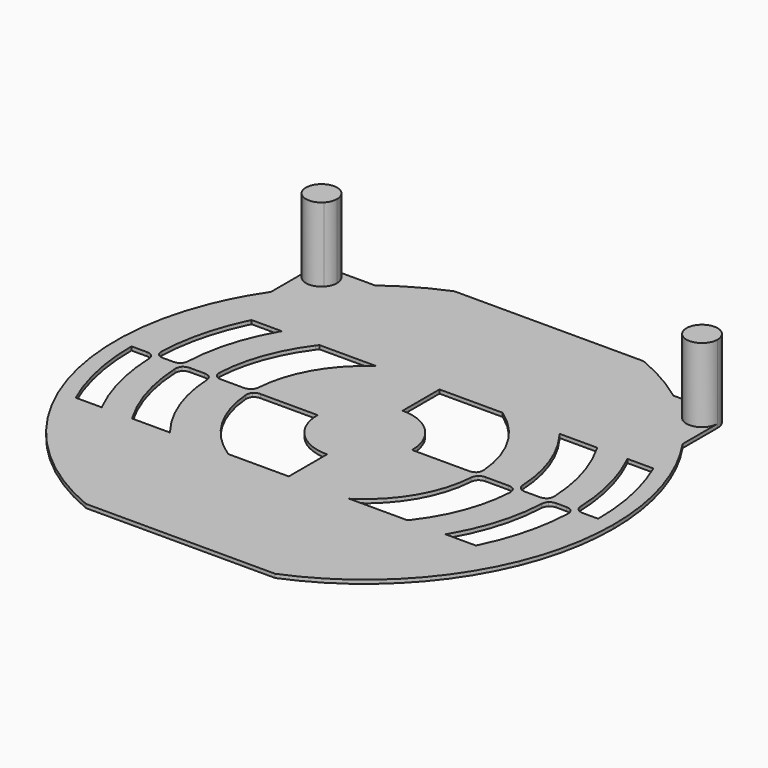
from build123d import *

# Parameters (mm, degrees)
F1_DEPTH    = 1.524
F2_T1_DEPTH = 1.524
F3_DEPTH    = 31.75
F5_DEPTH    = 12.7
F7_DEPTH    = 1.524


# Not quite as in the source:
# - a fillet or chamfer that OpenCascade refuses, or shapes differently, is made with other operations: its cross-section is extruded or revolved along the edge and cut away or added


with BuildPart() as f1:
    # F0 (on Top) → F1 (new body)
    with BuildSketch(Plane.XY):
        with BuildLine():
            ThreePointArc((-24.4320937034, 38.1), (-25.3223637573, 36.888098532), (-26.7450152278, 37.375283025))
            ThreePointArc((-26.7450152278, 37.375283025), (-40.5798224291, 21.5751160452), (-45.9412127468, 1.2698787713))
            ThreePointArc((-45.9412127468, 1.2698787713), (-45.0545517796, 0.8918001425), (-44.68876, 0))
            Line((-44.68876, 0), (-19.28622, 0))
            ThreePointArc((-19.28622, 0), (-13.6374169455, 13.6374169455), (0, 19.28622))
            Line((0, 19.28622), (0, 38.1))
            Line((0, 38.1), (-24.4320937034, 38.1))
        make_face()
        with BuildLine():
            ThreePointArc((25.7042798944, -38.0985251138), (40.2784862154, -22.1325816147), (45.9412127468, -1.2698787713))
            ThreePointArc((45.9412127468, -1.2698787713), (45.0545517796, -0.8918001425), (44.68876, 0))
            Line((44.68876, 0), (19.28622, 0))
            ThreePointArc((19.28622, 0), (13.6374169455, -13.6374169455), (0, -19.28622))
            Line((0, -19.28622), (0, -38.7942095688))
            Line((0, -38.7942095688), (23.3717719467, -38.7942095688))
            ThreePointArc((23.3717719467, -38.7942095688), (24.2787878517, -37.5771875695), (25.7042798944, -38.0985251138))
        make_face()
        with BuildLine():
            ThreePointArc((62.0544468751, 1.2699335332), (58.7091041954, 20.1397167987), (49.7668110589, 37.0895082899))
            ThreePointArc((49.7668110589, 37.0895082899), (48.4336499231, 36.9620417836), (47.7275214491, 38.1))
            Line((47.7275214491, 38.1), (26.9720937034, 38.1))
            ThreePointArc((26.9720937034, 38.1), (26.9139951713, 37.7202700539), (26.7450152278, 37.375283025))
            ThreePointArc((26.7450152278, 37.375283025), (40.5798224291, 21.5751160452), (45.9412127468, 1.2698787713))
            ThreePointArc((45.9412127468, 1.2698787713), (46.8505601425, 0.9042082204), (47.22876, 0))
            Line((47.22876, 0), (60.79744, 0))
            ThreePointArc((60.79744, 0), (61.1648323143, 0.8934200388), (62.0544468751, 1.2699335332))
        make_face()
        with BuildLine():
            ThreePointArc((64.5828161079, -37.7029056116), (72.0192608927, -20.1413824863), (74.7718960859, -1.2699542146))
            ThreePointArc((74.7718960859, -1.2699542146), (73.8808497579, -0.8942047945), (73.51268, 0))
            Line((73.51268, 0), (63.33744, 0))
            ThreePointArc((63.33744, 0), (62.9608600388, -0.9026076857), (62.0544468751, -1.2699335332))
            ThreePointArc((62.0544468751, -1.2699335332), (58.5641437485, -20.5574360064), (49.2333389626, -37.7947806284))
            ThreePointArc((49.2333389626, -37.7947806284), (49.5916770074, -38.238458905), (49.7197307741, -38.7942095688))
            Line((49.7197307741, -38.7942095688), (62.6632349558, -38.7942095688))
            ThreePointArc((62.6632349558, -38.7942095688), (63.3055678717, -37.6901561138), (64.5828161079, -37.7029056116))
        make_face()
        with BuildLine():
            ThreePointArc((85.6190619886, 1.2699650787), (83.3626938013, 19.5677762992), (77.2418743801, 36.9584825088))
            ThreePointArc((77.2418743801, 36.9584825088), (76.0121986911, 37.0230085698), (75.4152436073, 38.1))
            Line((75.4152436073, 38.1), (65.6193529725, 38.1))
            ThreePointArc((65.6193529725, 38.1), (65.4499936503, 37.4663675367), (64.9870851009, 37.0017296633))
            ThreePointArc((64.9870851009, 37.0017296633), (72.127201178, 19.7513563639), (74.7718960859, 1.2699542146))
            ThreePointArc((74.7718960859, 1.2699542146), (75.6768847945, 0.9018302421), (76.05268, 0))
            Line((76.05268, 0), (84.35848, 0))
            ThreePointArc((84.35848, 0), (84.7271307684, 0.8946896461), (85.6190619886, 1.2699650787))
        make_face()
        with BuildLine():
            ThreePointArc((93.901913207, -38.7942095688), (99.6568973575, -19.7753080655), (101.6, 0))
            Line((101.6, 0), (86.89848, 0))
            ThreePointArc((86.89848, 0), (86.5231696461, -0.9013492316), (85.6190619886, -1.2699650787))
            ThreePointArc((85.6190619886, -1.2699650787), (83.2730642114, -19.9457605507), (76.9033645528, -37.6577894674))
            ThreePointArc((76.9033645528, -37.6577894674), (77.4164332183, -38.1260574891), (77.6063995159, -38.7942095688))
            Line((77.6063995159, -38.7942095688), (93.901913207, -38.7942095688))
        make_face()
        with BuildLine():
            ThreePointArc((-60.79744, 0), (-61.1648323143, -0.8934200388), (-62.0544468751, -1.2699335332))
            ThreePointArc((-62.0544468751, -1.2699335332), (-58.5641437485, -20.5574360064), (-49.2333389626, -37.7947806284))
            ThreePointArc((-49.2333389626, -37.7947806284), (-47.8939801103, -37.6522633355), (-47.1797307741, -38.7942095688))
            Line((-47.1797307741, -38.7942095688), (-25.9117719467, -38.7942095688))
            ThreePointArc((-25.9117719467, -38.7942095688), (-25.858793946, -38.4312254739), (-25.7042798944, -38.0985251138))
            ThreePointArc((-25.7042798944, -38.0985251138), (-40.2784862154, -22.1325816147), (-45.9412127468, -1.2698787713))
            ThreePointArc((-45.9412127468, -1.2698787713), (-46.8505601425, -0.9042082204), (-47.22876, 0))
            Line((-47.22876, 0), (-60.79744, 0))
        make_face()
        with BuildLine():
            ThreePointArc((-62.6632349558, 38.1), (-63.4645367133, 36.9196517643), (-64.8572852825, 37.2287761518))
            ThreePointArc((-64.8572852825, 37.2287761518), (-72.0925536459, 19.8774479449), (-74.7718960859, 1.2699542146))
            ThreePointArc((-74.7718960859, 1.2699542146), (-73.8808497579, 0.8942047945), (-73.51268, 0))
            Line((-73.51268, 0), (-63.33744, 0))
            ThreePointArc((-63.33744, 0), (-62.9608600388, 0.9026076857), (-62.0544468751, 1.2699335332))
            ThreePointArc((-62.0544468751, 1.2699335332), (-58.7091041954, 20.1397167987), (-49.7668110589, 37.0895082899))
            ThreePointArc((-49.7668110589, 37.0895082899), (-50.1354796655, 37.536128474), (-50.2675214491, 38.1))
            Line((-50.2675214491, 38.1), (-62.6632349558, 38.1))
        make_face()
        with BuildLine():
            ThreePointArc((-84.35848, 0), (-84.7271307684, -0.8946896461), (-85.6190619886, -1.2699650787))
            ThreePointArc((-85.6190619886, -1.2699650787), (-83.2730642114, -19.9457605507), (-76.9033645528, -37.6577894674))
            ThreePointArc((-76.9033645528, -37.6577894674), (-75.6682474362, -37.7141758663), (-75.0663995159, -38.7942095688))
            Line((-75.0663995159, -38.7942095688), (-65.2032349558, -38.7942095688))
            ThreePointArc((-65.2032349558, -38.7942095688), (-65.0372884108, -38.1665424847), (-64.5828161079, -37.7029056116))
            ThreePointArc((-64.5828161079, -37.7029056116), (-72.0192608927, -20.1413824863), (-74.7718960859, -1.2699542146))
            ThreePointArc((-74.7718960859, -1.2699542146), (-75.6768847945, -0.9018302421), (-76.05268, 0))
            Line((-76.05268, 0), (-84.35848, 0))
        make_face()
        with BuildLine():
            Line((-77.9552436073, 38.1), (-94.1857207861, 38.1))
            ThreePointArc((-94.1857207861, 38.1), (-99.7292064339, 19.4073538656), (-101.6, 0))
            Line((-101.6, 0), (-86.89848, 0))
            ThreePointArc((-86.89848, 0), (-86.5231696461, 0.9013492316), (-85.6190619886, 1.2699650787))
            ThreePointArc((-85.6190619886, 1.2699650787), (-83.3626938013, 19.5677762992), (-77.2418743801, 36.9584825088))
            ThreePointArc((-77.2418743801, 36.9584825088), (-77.7622350375, 37.4269550838), (-77.9552436073, 38.1))
        make_face()
        with BuildLine():
            ThreePointArc((-85.6190619886, 1.2699650787), (-85.6261254648, 0.635), (-85.62848, 0))
            Line((-85.62848, 0), (-84.35848, 0))
            ThreePointArc((-84.35848, 0), (-84.7271307684, 0.8946896461), (-85.6190619886, 1.2699650787))
        make_face()
        with BuildLine():
            Line((-84.35848, 0), (-85.62848, 0))
            ThreePointArc((-85.62848, 0), (-85.6261254648, -0.635), (-85.6190619886, -1.2699650787))
            ThreePointArc((-85.6190619886, -1.2699650787), (-84.7271307684, -0.8946896461), (-84.35848, 0))
        make_face()
        with BuildLine():
            Line((-85.62848, 0), (-86.89848, 0))
            ThreePointArc((-86.89848, 0), (-86.5231696461, -0.9013492316), (-85.6190619886, -1.2699650787))
            ThreePointArc((-85.6190619886, -1.2699650787), (-85.6261254648, -0.635), (-85.62848, 0))
        make_face()
        with BuildLine():
            ThreePointArc((-85.6190619886, 1.2699650787), (-86.5231696461, 0.9013492316), (-86.89848, 0))
            Line((-86.89848, 0), (-85.62848, 0))
            ThreePointArc((-85.62848, 0), (-85.6261254648, 0.635), (-85.6190619886, 1.2699650787))
        make_face()
        with BuildLine():
            ThreePointArc((-74.7718960859, 1.2699542146), (-75.6768847945, 0.9018302421), (-76.05268, 0))
            Line((-76.05268, 0), (-74.78268, 0))
            ThreePointArc((-74.78268, 0), (-74.7799839729, 0.635), (-74.7718960859, 1.2699542146))
        make_face()
        with BuildLine():
            ThreePointArc((-74.7718960859, 1.2699542146), (-74.7799839729, 0.635), (-74.78268, 0))
            Line((-74.78268, 0), (-73.51268, 0))
            ThreePointArc((-73.51268, 0), (-73.8808497579, 0.8942047945), (-74.7718960859, 1.2699542146))
        make_face()
        with BuildLine():
            Line((-73.51268, 0), (-74.78268, 0))
            ThreePointArc((-74.78268, 0), (-74.7799839729, -0.635), (-74.7718960859, -1.2699542146))
            ThreePointArc((-74.7718960859, -1.2699542146), (-73.8808497579, -0.8942047945), (-73.51268, 0))
        make_face()
        with BuildLine():
            Line((-74.78268, 0), (-76.05268, 0))
            ThreePointArc((-76.05268, 0), (-75.6768847945, -0.9018302421), (-74.7718960859, -1.2699542146))
            ThreePointArc((-74.7718960859, -1.2699542146), (-74.7799839729, -0.635), (-74.78268, 0))
        make_face()
        with BuildLine():
            ThreePointArc((-62.0544468751, 1.2699335332), (-62.9608600388, 0.9026076857), (-63.33744, 0))
            Line((-63.33744, 0), (-62.06744, 0))
            ThreePointArc((-62.06744, 0), (-62.0641916338, 0.635), (-62.0544468751, 1.2699335332))
        make_face()
        with BuildLine():
            ThreePointArc((-62.0544468751, 1.2699335332), (-62.0641916338, 0.635), (-62.06744, 0))
            Line((-62.06744, 0), (-60.79744, 0))
            ThreePointArc((-60.79744, 0), (-61.1648323143, 0.8934200388), (-62.0544468751, 1.2699335332))
        make_face()
        with BuildLine():
            Line((-60.79744, 0), (-62.06744, 0))
            ThreePointArc((-62.06744, 0), (-62.0641916338, -0.635), (-62.0544468751, -1.2699335332))
            ThreePointArc((-62.0544468751, -1.2699335332), (-61.1648323143, -0.8934200388), (-60.79744, 0))
        make_face()
        with BuildLine():
            Line((-62.06744, 0), (-63.33744, 0))
            ThreePointArc((-63.33744, 0), (-62.9608600388, -0.9026076857), (-62.0544468751, -1.2699335332))
            ThreePointArc((-62.0544468751, -1.2699335332), (-62.0641916338, -0.635), (-62.06744, 0))
        make_face()
        with BuildLine():
            ThreePointArc((-45.9412127468, 1.2698787713), (-46.8505601425, 0.9042082204), (-47.22876, 0))
            Line((-47.22876, 0), (-45.95876, 0))
            ThreePointArc((-45.95876, 0), (-45.9543729773, 0.635), (-45.9412127468, 1.2698787713))
        make_face()
        with BuildLine():
            ThreePointArc((-45.9412127468, 1.2698787713), (-45.9543729773, 0.635), (-45.95876, 0))
            Line((-45.95876, 0), (-44.68876, 0))
            ThreePointArc((-44.68876, 0), (-45.0545517796, 0.8918001425), (-45.9412127468, 1.2698787713))
        make_face()
        with BuildLine():
            Line((-44.68876, 0), (-45.95876, 0))
            ThreePointArc((-45.95876, 0), (-45.9543729773, -0.635), (-45.9412127468, -1.2698787713))
            ThreePointArc((-45.9412127468, -1.2698787713), (-45.0545517796, -0.8918001425), (-44.68876, 0))
        make_face()
        with BuildLine():
            Line((-45.95876, 0), (-47.22876, 0))
            ThreePointArc((-47.22876, 0), (-46.8505601425, -0.9042082204), (-45.9412127468, -1.2698787713))
            ThreePointArc((-45.9412127468, -1.2698787713), (-45.9543729773, -0.635), (-45.95876, 0))
        make_face()
        with BuildLine():
            ThreePointArc((45.9412127468, -1.2698787713), (46.8505601425, -0.9042082204), (47.22876, 0))
            Line((47.22876, 0), (45.95876, 0))
            ThreePointArc((45.95876, 0), (45.9543729773, -0.635), (45.9412127468, -1.2698787713))
        make_face()
        with BuildLine():
            Line((45.95876, 0), (47.22876, 0))
            ThreePointArc((47.22876, 0), (46.8505601425, 0.9042082204), (45.9412127468, 1.2698787713))
            ThreePointArc((45.9412127468, 1.2698787713), (45.9543729773, 0.635), (45.95876, 0))
        make_face()
        with BuildLine():
            Line((44.68876, 0), (45.95876, 0))
            ThreePointArc((45.95876, 0), (45.9543729773, 0.635), (45.9412127468, 1.2698787713))
            ThreePointArc((45.9412127468, 1.2698787713), (45.0545517796, 0.8918001425), (44.68876, 0))
        make_face()
        with BuildLine():
            Line((60.79744, 0), (62.06744, 0))
            ThreePointArc((62.06744, 0), (62.0641916338, 0.635), (62.0544468751, 1.2699335332))
            ThreePointArc((62.0544468751, 1.2699335332), (61.1648323143, 0.8934200388), (60.79744, 0))
        make_face()
        with BuildLine():
            Line((62.06744, 0), (63.33744, 0))
            ThreePointArc((63.33744, 0), (62.9608600388, 0.9026076857), (62.0544468751, 1.2699335332))
            ThreePointArc((62.0544468751, 1.2699335332), (62.0641916338, 0.635), (62.06744, 0))
        make_face()
        with BuildLine():
            ThreePointArc((62.0544468751, -1.2699335332), (62.9608600388, -0.9026076857), (63.33744, 0))
            Line((63.33744, 0), (62.06744, 0))
            ThreePointArc((62.06744, 0), (62.0641916338, -0.635), (62.0544468751, -1.2699335332))
        make_face()
        with BuildLine():
            ThreePointArc((62.0544468751, -1.2699335332), (62.0641916338, -0.635), (62.06744, 0))
            Line((62.06744, 0), (60.79744, 0))
            ThreePointArc((60.79744, 0), (61.1648323143, -0.8934200388), (62.0544468751, -1.2699335332))
        make_face()
        with BuildLine():
            Line((73.51268, 0), (74.78268, 0))
            ThreePointArc((74.78268, 0), (74.7799839729, 0.635), (74.7718960859, 1.2699542146))
            ThreePointArc((74.7718960859, 1.2699542146), (73.8808497579, 0.8942047945), (73.51268, 0))
        make_face()
        with BuildLine():
            ThreePointArc((74.7718960859, -1.2699542146), (74.7799839729, -0.635), (74.78268, 0))
            Line((74.78268, 0), (73.51268, 0))
            ThreePointArc((73.51268, 0), (73.8808497579, -0.8942047945), (74.7718960859, -1.2699542146))
        make_face()
        with BuildLine():
            ThreePointArc((74.7718960859, -1.2699542146), (75.6768847945, -0.9018302421), (76.05268, 0))
            Line((76.05268, 0), (74.78268, 0))
            ThreePointArc((74.78268, 0), (74.7799839729, -0.635), (74.7718960859, -1.2699542146))
        make_face()
        with BuildLine():
            Line((74.78268, 0), (76.05268, 0))
            ThreePointArc((76.05268, 0), (75.6768847945, 0.9018302421), (74.7718960859, 1.2699542146))
            ThreePointArc((74.7718960859, 1.2699542146), (74.7799839729, 0.635), (74.78268, 0))
        make_face()
        with BuildLine():
            Line((84.35848, 0), (85.62848, 0))
            ThreePointArc((85.62848, 0), (85.6261254648, 0.635), (85.6190619886, 1.2699650787))
            ThreePointArc((85.6190619886, 1.2699650787), (84.7271307684, 0.8946896461), (84.35848, 0))
        make_face()
        with BuildLine():
            Line((85.62848, 0), (86.89848, 0))
            ThreePointArc((86.89848, 0), (86.5231696461, 0.9013492316), (85.6190619886, 1.2699650787))
            ThreePointArc((85.6190619886, 1.2699650787), (85.6261254648, 0.635), (85.62848, 0))
        make_face()
        with BuildLine():
            ThreePointArc((85.6190619886, -1.2699650787), (86.5231696461, -0.9013492316), (86.89848, 0))
            Line((86.89848, 0), (85.62848, 0))
            ThreePointArc((85.62848, 0), (85.6261254648, -0.635), (85.6190619886, -1.2699650787))
        make_face()
        with BuildLine():
            ThreePointArc((85.6190619886, -1.2699650787), (85.6261254648, -0.635), (85.62848, 0))
            Line((85.62848, 0), (84.35848, 0))
            ThreePointArc((84.35848, 0), (84.7271307684, -0.8946896461), (85.6190619886, -1.2699650787))
        make_face()
        with BuildLine():
            Line((0, 0), (0, 19.28622))
            ThreePointArc((0, 19.28622), (-13.6374169455, 13.6374169455), (-19.28622, 0))
            Line((-19.28622, 0), (0, 0))
        make_face()
        with BuildLine():
            Line((0, 0), (19.28622, 0))
            ThreePointArc((19.28622, 0), (13.6374169455, 13.6374169455), (0, 19.28622))
            Line((0, 19.28622), (0, 0))
        make_face()
        with BuildLine():
            ThreePointArc((0, -19.28622), (13.6374169455, -13.6374169455), (19.28622, 0))
            Line((19.28622, 0), (0, 0))
            Line((0, 0), (0, -19.28622))
        make_face()
        with BuildLine():
            Line((0, 0), (-19.28622, 0))
            ThreePointArc((-19.28622, 0), (-13.6374169455, -13.6374169455), (0, -19.28622))
            Line((0, -19.28622), (0, 0))
        make_face()
        with BuildLine():
            ThreePointArc((45.9412127468, -1.2698787713), (45.9543729773, -0.635), (45.95876, 0))
            Line((45.95876, 0), (44.68876, 0))
            ThreePointArc((44.68876, 0), (45.0545517796, -0.8918001425), (45.9412127468, -1.2698787713))
        make_face()
        with BuildLine():
            ThreePointArc((73.0914093882, 70.5705737092), (67.2072279768, 76.1954625137), (60.8916274027, 81.3312345428))
            ThreePointArc((60.8916274027, 81.3312345428), (0, 101.6), (-60.8916274027, 81.3312345428))
            ThreePointArc((-60.8916274027, 81.3312345428), (-67.2072281578, 76.195462354), (-73.0914097236, 70.5705733618))
            ThreePointArc((-73.0914097236, 70.5705733618), (-78.8370521258, 64.0880582646), (-84.0096224974, 57.1396826019))
            ThreePointArc((-84.0096224974, 57.1396826019), (-89.6048127635, 47.8908919276), (-94.1857207861, 38.1))
            Line((-94.1857207861, 38.1), (-77.9552436073, 38.1))
            ThreePointArc((-77.9552436073, 38.1), (-77.35028331, 39.1819529536), (-76.1117440894, 39.2331364891))
            ThreePointArc((-76.1117440894, 39.2331364891), (0, 85.62848), (76.1117440894, 39.2331364891))
            ThreePointArc((76.1117440894, 39.2331364891), (77.35028331, 39.1819529536), (77.9552436073, 38.1))
            Line((77.9552436073, 38.1), (94.1857207861, 38.1))
            ThreePointArc((94.1857207861, 38.1), (89.6048127635, 47.8908919276), (84.0096224974, 57.1396826019))
            ThreePointArc((84.0096224974, 57.1396826019), (78.8370519734, 64.0880584519), (73.0914093882, 70.5705737092))
        make_face()
        with BuildLine():
            ThreePointArc((75.4152436073, 38.1), (75.6032906537, 38.7650397027), (76.1117440894, 39.2331364891))
            ThreePointArc((76.1117440894, 39.2331364891), (0, 85.62848), (-76.1117440894, 39.2331364891))
            ThreePointArc((-76.1117440894, 39.2331364891), (-75.6032906537, 38.7650397027), (-75.4152436073, 38.1))
            Line((-75.4152436073, 38.1), (-65.2032349558, 38.1))
            ThreePointArc((-65.2032349558, 38.1), (-64.7072509575, 39.106875975), (-63.6067007367, 39.3273041203))
            ThreePointArc((-63.6067007367, 39.3273041203), (0.0822563989, 74.7826347615), (63.6930620577, 39.1872820403))
            ThreePointArc((63.6930620577, 39.1872820403), (64.9736167542, 39.2059813429), (65.6193529725, 38.1))
            Line((65.6193529725, 38.1), (75.4152436073, 38.1))
        make_face()
        with BuildLine():
            ThreePointArc((63.0793529725, 38.1), (63.2433716296, 38.7242637816), (63.6930620577, 39.1872820403))
            ThreePointArc((63.6930620577, 39.1872820403), (0.0822563989, 74.7826347615), (-63.6067007367, 39.3273041203))
            ThreePointArc((-63.6067007367, 39.3273041203), (-62.9263589808, 38.8740160017), (-62.6632349558, 38.1))
            Line((-62.6632349558, 38.1), (-50.2675214491, 38.1))
            ThreePointArc((-50.2675214491, 38.1), (-49.5497212333, 39.2436675209), (-48.2077176723, 39.0945400918))
            ThreePointArc((-48.2077176723, 39.0945400918), (0, 62.06744), (48.2077176723, 39.0945400918))
            ThreePointArc((48.2077176723, 39.0945400918), (49.5497212333, 39.2436675209), (50.2675214491, 38.1))
            Line((50.2675214491, 38.1), (63.0793529725, 38.1))
        make_face()
        with BuildLine():
            ThreePointArc((47.7275214491, 38.1), (47.8538539282, 38.6521997842), (48.2077176723, 39.0945400918))
            ThreePointArc((48.2077176723, 39.0945400918), (0, 62.06744), (-48.2077176723, 39.0945400918))
            ThreePointArc((-48.2077176723, 39.0945400918), (-47.8538539282, 38.6521997842), (-47.7275214491, 38.1))
            Line((-47.7275214491, 38.1), (-26.9720937034, 38.1))
            ThreePointArc((-26.9720937034, 38.1), (-26.0650428809, 39.3170324131), (-24.639545838, 38.7956234856))
            ThreePointArc((-24.639545838, 38.7956234856), (0, 45.95876), (24.639545838, 38.7956234856))
            ThreePointArc((24.639545838, 38.7956234856), (26.0650428809, 39.3170324131), (26.9720937034, 38.1))
            Line((26.9720937034, 38.1), (47.7275214491, 38.1))
        make_face()
        with BuildLine():
            ThreePointArc((24.4320937034, 38.1), (24.4850612903, 38.4629491775), (24.639545838, 38.7956234856))
            ThreePointArc((24.639545838, 38.7956234856), (0, 45.95876), (-24.639545838, 38.7956234856))
            ThreePointArc((-24.639545838, 38.7956234856), (-24.4850612903, 38.4629491775), (-24.4320937034, 38.1))
            Line((-24.4320937034, 38.1), (0, 38.1))
            Line((0, 38.1), (24.4320937034, 38.1))
        make_face()
        with BuildLine():
            ThreePointArc((-23.5604473288, -39.46027043), (0, -45.95876), (23.5604473288, -39.46027043))
            ThreePointArc((23.5604473288, -39.46027043), (23.419850864, -39.1403437446), (23.3717719467, -38.7942095688))
            Line((23.3717719467, -38.7942095688), (0, -38.7942095688))
            Line((0, -38.7942095688), (-23.3717719467, -38.7942095688))
            ThreePointArc((-23.3717719467, -38.7942095688), (-23.419850864, -39.1403437446), (-23.5604473288, -39.46027043))
        make_face()
        with BuildLine():
            ThreePointArc((-63.2652150285, -39.8743250148), (0, -74.78268), (63.2652150285, -39.8743250148))
            ThreePointArc((63.2652150285, -39.8743250148), (62.8238916123, -39.4124792075), (62.6632349558, -38.7942095688))
            Line((62.6632349558, -38.7942095688), (49.7197307741, -38.7942095688))
            ThreePointArc((49.7197307741, -38.7942095688), (48.9937693206, -39.9417818149), (47.6458377663, -39.7773962408))
            ThreePointArc((47.6458377663, -39.7773962408), (0, -62.06744), (-47.6458377663, -39.7773962408))
            ThreePointArc((-47.6458377663, -39.7773962408), (-48.9937693206, -39.9417818149), (-49.7197307741, -38.7942095688))
            Line((-49.7197307741, -38.7942095688), (-62.6632349558, -38.7942095688))
            ThreePointArc((-62.6632349558, -38.7942095688), (-62.8238916123, -39.4124792075), (-63.2652150285, -39.8743250148))
        make_face()
        with BuildLine():
            ThreePointArc((-75.7526424704, -39.9220959602), (0, -85.62848), (75.7526424704, -39.9220959602))
            ThreePointArc((75.7526424704, -39.9220959602), (75.2514406577, -39.4543340087), (75.0663995159, -38.7942095688))
            Line((75.0663995159, -38.7942095688), (65.2032349558, -38.7942095688))
            ThreePointArc((65.2032349558, -38.7942095688), (64.5515045945, -39.9035529123), (63.2652150285, -39.8743250148))
            ThreePointArc((63.2652150285, -39.8743250148), (0, -74.78268), (-63.2652150285, -39.8743250148))
            ThreePointArc((-63.2652150285, -39.8743250148), (-64.5515045945, -39.9035529123), (-65.2032349558, -38.7942095688))
            Line((-65.2032349558, -38.7942095688), (-75.0663995159, -38.7942095688))
            ThreePointArc((-75.0663995159, -38.7942095688), (-75.2514406577, -39.4543340087), (-75.7526424704, -39.9220959602))
        make_face()
        with BuildLine():
            ThreePointArc((-93.901913207, -38.7942095688), (0, -101.6), (93.901913207, -38.7942095688))
            Line((93.901913207, -38.7942095688), (77.6063995159, -38.7942095688))
            ThreePointArc((77.6063995159, -38.7942095688), (76.9965239558, -39.8791684269), (75.7526424704, -39.9220959602))
            ThreePointArc((75.7526424704, -39.9220959602), (0, -85.62848), (-75.7526424704, -39.9220959602))
            ThreePointArc((-75.7526424704, -39.9220959602), (-76.9965239558, -39.8791684269), (-77.6063995159, -38.7942095688))
            Line((-77.6063995159, -38.7942095688), (-93.901913207, -38.7942095688))
        make_face()
        with BuildLine():
            ThreePointArc((26.7450152278, 37.375283025), (26.9139951713, 37.7202700539), (26.9720937034, 38.1))
            Line((26.9720937034, 38.1), (25.7020937034, 38.1))
            ThreePointArc((25.7020937034, 38.1), (26.2260578907, 37.741244127), (26.7450152278, 37.375283025))
        make_face()
        with BuildLine():
            Line((24.4320937034, 38.1), (25.7020937034, 38.1))
            ThreePointArc((25.7020937034, 38.1), (25.1732226967, 38.4514821535), (24.639545838, 38.7956234856))
            ThreePointArc((24.639545838, 38.7956234856), (24.4850612903, 38.4629491775), (24.4320937034, 38.1))
        make_face()
        with BuildLine():
            ThreePointArc((-24.639545838, 38.7956234856), (-26.0650428809, 39.3170324131), (-26.9720937034, 38.1))
            Line((-26.9720937034, 38.1), (-25.7020937034, 38.1))
            ThreePointArc((-25.7020937034, 38.1), (-25.1732226967, 38.4514821535), (-24.639545838, 38.7956234856))
        make_face()
        with BuildLine():
            ThreePointArc((-24.639545838, 38.7956234856), (-25.1732226967, 38.4514821535), (-25.7020937034, 38.1))
            Line((-25.7020937034, 38.1), (-24.4320937034, 38.1))
            ThreePointArc((-24.4320937034, 38.1), (-24.4850612903, 38.4629491775), (-24.639545838, 38.7956234856))
        make_face()
        with BuildLine():
            ThreePointArc((-25.7042798944, -38.0985251138), (-25.858793946, -38.4312254739), (-25.9117719467, -38.7942095688))
            Line((-25.9117719467, -38.7942095688), (-24.6417719467, -38.7942095688))
            ThreePointArc((-24.6417719467, -38.7942095688), (-25.1754290572, -38.4500376141), (-25.7042798944, -38.0985251138))
        make_face()
        with BuildLine():
            Line((-23.3717719467, -38.7942095688), (-24.6417719467, -38.7942095688))
            ThreePointArc((-24.6417719467, -38.7942095688), (-24.1034104441, -39.1309752715), (-23.5604473288, -39.46027043))
            ThreePointArc((-23.5604473288, -39.46027043), (-23.419850864, -39.1403437446), (-23.3717719467, -38.7942095688))
        make_face()
        with BuildLine():
            ThreePointArc((23.5604473288, -39.46027043), (24.1034104441, -39.1309752715), (24.6417719467, -38.7942095688))
            Line((24.6417719467, -38.7942095688), (23.3717719467, -38.7942095688))
            ThreePointArc((23.3717719467, -38.7942095688), (23.419850864, -39.1403437446), (23.5604473288, -39.46027043))
        make_face()
        with BuildLine():
            ThreePointArc((23.5604473288, -39.46027043), (24.9879061224, -40.0161306515), (25.9117719467, -38.7942095688))
            Line((25.9117719467, -38.7942095688), (24.6417719467, -38.7942095688))
            ThreePointArc((24.6417719467, -38.7942095688), (24.1034104441, -39.1309752715), (23.5604473288, -39.46027043))
        make_face()
        with BuildLine():
            Line((23.3717719467, -38.7942095688), (24.6417719467, -38.7942095688))
            ThreePointArc((24.6417719467, -38.7942095688), (25.1754290571, -38.4500376141), (25.7042798944, -38.0985251138))
            ThreePointArc((25.7042798944, -38.0985251138), (24.2787878517, -37.5771875695), (23.3717719467, -38.7942095688))
        make_face()
        with BuildLine():
            ThreePointArc((-47.6458377663, -39.7773962408), (0, -62.06744), (47.6458377663, -39.7773962408))
            ThreePointArc((47.6458377663, -39.7773962408), (47.3021585281, -39.3382481153), (47.1797307741, -38.7942095688))
            Line((47.1797307741, -38.7942095688), (25.9117719467, -38.7942095688))
            ThreePointArc((25.9117719467, -38.7942095688), (24.9879061224, -40.0161306515), (23.5604473288, -39.46027043))
            ThreePointArc((23.5604473288, -39.46027043), (0, -45.95876), (-23.5604473288, -39.46027043))
            ThreePointArc((-23.5604473288, -39.46027043), (-24.9879061224, -40.0161306515), (-25.9117719467, -38.7942095688))
            Line((-25.9117719467, -38.7942095688), (-47.1797307741, -38.7942095688))
            ThreePointArc((-47.1797307741, -38.7942095688), (-47.3021585281, -39.3382481153), (-47.6458377663, -39.7773962408))
        make_face()
        with BuildLine():
            Line((-24.6417719467, -38.7942095688), (-25.9117719467, -38.7942095688))
            ThreePointArc((-25.9117719467, -38.7942095688), (-24.9879061224, -40.0161306515), (-23.5604473288, -39.46027043))
            ThreePointArc((-23.5604473288, -39.46027043), (-24.1034104441, -39.1309752715), (-24.6417719467, -38.7942095688))
        make_face()
        with BuildLine():
            ThreePointArc((47.6458377663, -39.7773962408), (48.0502990343, -39.2878590771), (48.4497307741, -38.7942095688))
            Line((48.4497307741, -38.7942095688), (47.1797307741, -38.7942095688))
            ThreePointArc((47.1797307741, -38.7942095688), (47.3021585281, -39.3382481153), (47.6458377663, -39.7773962408))
        make_face()
        with BuildLine():
            ThreePointArc((47.6458377663, -39.7773962408), (48.9937693206, -39.9417818149), (49.7197307741, -38.7942095688))
            Line((49.7197307741, -38.7942095688), (48.4497307741, -38.7942095688))
            ThreePointArc((48.4497307741, -38.7942095688), (48.0502990343, -39.2878590771), (47.6458377663, -39.7773962408))
        make_face()
        with BuildLine():
            Line((48.4497307741, -38.7942095688), (49.7197307741, -38.7942095688))
            ThreePointArc((49.7197307741, -38.7942095688), (49.5916770074, -38.238458905), (49.2333389626, -37.7947806284))
            ThreePointArc((49.2333389626, -37.7947806284), (48.8440911764, -38.2964993871), (48.4497307741, -38.7942095688))
        make_face()
        with BuildLine():
            ThreePointArc((63.2652150285, -39.8743250148), (63.6015179217, -39.3356854019), (63.9332349558, -38.7942095688))
            Line((63.9332349558, -38.7942095688), (62.6632349558, -38.7942095688))
            ThreePointArc((62.6632349558, -38.7942095688), (62.8238916123, -39.4124792075), (63.2652150285, -39.8743250148))
        make_face()
        with BuildLine():
            Line((62.6632349558, -38.7942095688), (63.9332349558, -38.7942095688))
            ThreePointArc((63.9332349558, -38.7942095688), (64.260342213, -38.2499365575), (64.5828161079, -37.7029056116))
            ThreePointArc((64.5828161079, -37.7029056116), (63.3055678717, -37.6901561138), (62.6632349558, -38.7942095688))
        make_face()
        with BuildLine():
            ThreePointArc((63.2652150285, -39.8743250148), (64.5515045945, -39.9035529123), (65.2032349558, -38.7942095688))
            Line((65.2032349558, -38.7942095688), (63.9332349558, -38.7942095688))
            ThreePointArc((63.9332349558, -38.7942095688), (63.6015179217, -39.3356854019), (63.2652150285, -39.8743250148))
        make_face()
        with BuildLine():
            ThreePointArc((75.7526424704, -39.9220959602), (76.0466120547, -39.3592350295), (76.3363995159, -38.7942095688))
            Line((76.3363995159, -38.7942095688), (75.0663995159, -38.7942095688))
            ThreePointArc((75.0663995159, -38.7942095688), (75.2514406577, -39.4543340087), (75.7526424704, -39.9220959602))
        make_face()
        with BuildLine():
            ThreePointArc((75.7526424704, -39.9220959602), (76.9965239558, -39.8791684269), (77.6063995159, -38.7942095688))
            Line((77.6063995159, -38.7942095688), (76.3363995159, -38.7942095688))
            ThreePointArc((76.3363995159, -38.7942095688), (76.0466120547, -39.3592350295), (75.7526424704, -39.9220959602))
        make_face()
        with BuildLine():
            Line((76.3363995159, -38.7942095688), (77.6063995159, -38.7942095688))
            ThreePointArc((77.6063995159, -38.7942095688), (77.4164332183, -38.1260574891), (76.9033645528, -37.6577894674))
            ThreePointArc((76.9033645528, -37.6577894674), (76.6219889171, -38.2270506513), (76.3363995159, -38.7942095688))
        make_face()
        with BuildLine():
            Line((76.6852436073, 38.1), (77.9552436073, 38.1))
            ThreePointArc((77.9552436073, 38.1), (77.35028331, 39.1819529536), (76.1117440894, 39.2331364891))
            ThreePointArc((76.1117440894, 39.2331364891), (76.4005946435, 38.6676314925), (76.6852436073, 38.1))
        make_face()
        with BuildLine():
            Line((75.4152436073, 38.1), (76.6852436073, 38.1))
            ThreePointArc((76.6852436073, 38.1), (76.4005946435, 38.6676314925), (76.1117440894, 39.2331364891))
            ThreePointArc((76.1117440894, 39.2331364891), (75.6032906537, 38.7650397027), (75.4152436073, 38.1))
        make_face()
        with BuildLine():
            ThreePointArc((77.2418743801, 36.9584825088), (76.9656753269, 37.5302732282), (76.6852436073, 38.1))
            Line((76.6852436073, 38.1), (75.4152436073, 38.1))
            ThreePointArc((75.4152436073, 38.1), (76.0121986911, 37.0230085698), (77.2418743801, 36.9584825088))
        make_face()
        with BuildLine():
            ThreePointArc((64.9870851009, 37.0017296633), (65.4499936503, 37.4663675367), (65.6193529725, 38.1))
            Line((65.6193529725, 38.1), (64.3493529725, 38.1))
            ThreePointArc((64.3493529725, 38.1), (64.6705505065, 37.5522186451), (64.9870851009, 37.0017296633))
        make_face()
        with BuildLine():
            Line((64.3493529725, 38.1), (65.6193529725, 38.1))
            ThreePointArc((65.6193529725, 38.1), (64.9736167542, 39.2059813429), (63.6930620577, 39.1872820403))
            ThreePointArc((63.6930620577, 39.1872820403), (64.0235156583, 38.6450342312), (64.3493529725, 38.1))
        make_face()
        with BuildLine():
            Line((63.0793529725, 38.1), (64.3493529725, 38.1))
            ThreePointArc((64.3493529725, 38.1), (64.0235156583, 38.6450342312), (63.6930620577, 39.1872820403))
            ThreePointArc((63.6930620577, 39.1872820403), (63.2433716296, 38.7242637816), (63.0793529725, 38.1))
        make_face()
        with BuildLine():
            ThreePointArc((49.7668110589, 37.0895082899), (49.384750858, 37.5967218098), (48.9975214491, 38.1))
            Line((48.9975214491, 38.1), (47.7275214491, 38.1))
            ThreePointArc((47.7275214491, 38.1), (48.4336499231, 36.9620417836), (49.7668110589, 37.0895082899))
        make_face()
        with BuildLine():
            Line((47.7275214491, 38.1), (48.9975214491, 38.1))
            ThreePointArc((48.9975214491, 38.1), (48.6051633642, 38.5992901812), (48.2077176723, 39.0945400918))
            ThreePointArc((48.2077176723, 39.0945400918), (47.8538539282, 38.6521997842), (47.7275214491, 38.1))
        make_face()
        with BuildLine():
            Line((48.9975214491, 38.1), (50.2675214491, 38.1))
            ThreePointArc((50.2675214491, 38.1), (49.5497212333, 39.2436675209), (48.2077176723, 39.0945400918))
            ThreePointArc((48.2077176723, 39.0945400918), (48.6051633642, 38.5992901812), (48.9975214491, 38.1))
        make_face()
        with BuildLine():
            Line((25.7020937034, 38.1), (26.9720937034, 38.1))
            ThreePointArc((26.9720937034, 38.1), (26.0650428809, 39.3170324131), (24.639545838, 38.7956234856))
            ThreePointArc((24.639545838, 38.7956234856), (25.1732226967, 38.4514821535), (25.7020937034, 38.1))
        make_face()
        with BuildLine():
            Line((-24.4320937034, 38.1), (-25.7020937034, 38.1))
            ThreePointArc((-25.7020937034, 38.1), (-26.2260578907, 37.741244127), (-26.7450152278, 37.375283025))
            ThreePointArc((-26.7450152278, 37.375283025), (-25.3223637573, 36.888098532), (-24.4320937034, 38.1))
        make_face()
        with BuildLine():
            ThreePointArc((-48.2077176723, 39.0945400918), (-49.5497212333, 39.2436675209), (-50.2675214491, 38.1))
            Line((-50.2675214491, 38.1), (-48.9975214491, 38.1))
            ThreePointArc((-48.9975214491, 38.1), (-48.6051633642, 38.5992901812), (-48.2077176723, 39.0945400918))
        make_face()
        with BuildLine():
            ThreePointArc((-48.2077176723, 39.0945400918), (-48.6051633642, 38.5992901812), (-48.9975214491, 38.1))
            Line((-48.9975214491, 38.1), (-47.7275214491, 38.1))
            ThreePointArc((-47.7275214491, 38.1), (-47.8538539282, 38.6521997842), (-48.2077176723, 39.0945400918))
        make_face()
        with BuildLine():
            Line((-48.9975214491, 38.1), (-50.2675214491, 38.1))
            ThreePointArc((-50.2675214491, 38.1), (-50.1354796655, 37.536128474), (-49.7668110589, 37.0895082899))
            ThreePointArc((-49.7668110589, 37.0895082899), (-49.384750858, 37.5967218098), (-48.9975214491, 38.1))
        make_face()
        with BuildLine():
            ThreePointArc((-63.6067007367, 39.3273041203), (-64.7072509575, 39.106875975), (-65.2032349558, 38.1))
            Line((-65.2032349558, 38.1), (-64.3493529725, 38.1))
            ThreePointArc((-64.3493529725, 38.1), (-63.9809697415, 38.7154328262), (-63.6067007367, 39.3273041203))
        make_face()
        with BuildLine():
            ThreePointArc((-63.6067007367, 39.3273041203), (-63.9809697415, 38.7154328262), (-64.3493529725, 38.1))
            Line((-64.3493529725, 38.1), (-62.6632349558, 38.1))
            ThreePointArc((-62.6632349558, 38.1), (-62.9263589808, 38.8740160017), (-63.6067007367, 39.3273041203))
        make_face()
        with BuildLine():
            Line((-62.6632349558, 38.1), (-64.3493529725, 38.1))
            ThreePointArc((-64.3493529725, 38.1), (-64.6047877486, 37.6652442968), (-64.8572852825, 37.2287761518))
            ThreePointArc((-64.8572852825, 37.2287761518), (-63.4645367133, 36.9196517643), (-62.6632349558, 38.1))
        make_face()
        with BuildLine():
            Line((-76.6852436073, 38.1), (-77.9552436073, 38.1))
            ThreePointArc((-77.9552436073, 38.1), (-77.7622350375, 37.4269550838), (-77.2418743801, 36.9584825088))
            ThreePointArc((-77.2418743801, 36.9584825088), (-76.9656753269, 37.5302732282), (-76.6852436073, 38.1))
        make_face()
        with BuildLine():
            ThreePointArc((-76.1117440894, 39.2331364891), (-76.4005946435, 38.6676314925), (-76.6852436073, 38.1))
            Line((-76.6852436073, 38.1), (-75.4152436073, 38.1))
            ThreePointArc((-75.4152436073, 38.1), (-75.6032906537, 38.7650397027), (-76.1117440894, 39.2331364891))
        make_face()
        with BuildLine():
            Line((-48.4497307741, -38.7942095688), (-49.7197307741, -38.7942095688))
            ThreePointArc((-49.7197307741, -38.7942095688), (-48.9937693206, -39.9417818149), (-47.6458377663, -39.7773962408))
            ThreePointArc((-47.6458377663, -39.7773962408), (-48.0502990343, -39.2878590771), (-48.4497307741, -38.7942095688))
        make_face()
        with BuildLine():
            Line((-47.1797307741, -38.7942095688), (-48.4497307741, -38.7942095688))
            ThreePointArc((-48.4497307741, -38.7942095688), (-48.0502990343, -39.2878590771), (-47.6458377663, -39.7773962408))
            ThreePointArc((-47.6458377663, -39.7773962408), (-47.3021585281, -39.3382481153), (-47.1797307741, -38.7942095688))
        make_face()
        with BuildLine():
            ThreePointArc((-49.2333389626, -37.7947806284), (-48.8440911764, -38.2964993871), (-48.4497307741, -38.7942095688))
            Line((-48.4497307741, -38.7942095688), (-47.1797307741, -38.7942095688))
            ThreePointArc((-47.1797307741, -38.7942095688), (-47.8939801103, -37.6522633355), (-49.2333389626, -37.7947806284))
        make_face()
        with BuildLine():
            ThreePointArc((-64.5828161079, -37.7029056116), (-65.0372884108, -38.1665424847), (-65.2032349558, -38.7942095688))
            Line((-65.2032349558, -38.7942095688), (-63.9332349558, -38.7942095688))
            ThreePointArc((-63.9332349558, -38.7942095688), (-64.260342213, -38.2499365575), (-64.5828161079, -37.7029056116))
        make_face()
        with BuildLine():
            Line((-63.9332349558, -38.7942095688), (-65.2032349558, -38.7942095688))
            ThreePointArc((-65.2032349558, -38.7942095688), (-64.5515045945, -39.9035529123), (-63.2652150285, -39.8743250148))
            ThreePointArc((-63.2652150285, -39.8743250148), (-63.6015179217, -39.3356854019), (-63.9332349558, -38.7942095688))
        make_face()
        with BuildLine():
            Line((-62.6632349558, -38.7942095688), (-63.9332349558, -38.7942095688))
            ThreePointArc((-63.9332349558, -38.7942095688), (-63.6015179217, -39.3356854019), (-63.2652150285, -39.8743250148))
            ThreePointArc((-63.2652150285, -39.8743250148), (-62.8238916123, -39.4124792075), (-62.6632349558, -38.7942095688))
        make_face()
        with BuildLine():
            Line((-76.3363995159, -38.7942095688), (-77.6063995159, -38.7942095688))
            ThreePointArc((-77.6063995159, -38.7942095688), (-76.9965239558, -39.8791684269), (-75.7526424704, -39.9220959602))
            ThreePointArc((-75.7526424704, -39.9220959602), (-76.0466120547, -39.3592350295), (-76.3363995159, -38.7942095688))
        make_face()
        with BuildLine():
            Line((-75.0663995159, -38.7942095688), (-76.3363995159, -38.7942095688))
            ThreePointArc((-76.3363995159, -38.7942095688), (-76.0466120547, -39.3592350295), (-75.7526424704, -39.9220959602))
            ThreePointArc((-75.7526424704, -39.9220959602), (-75.2514406577, -39.4543340087), (-75.0663995159, -38.7942095688))
        make_face()
        with BuildLine():
            ThreePointArc((-76.9033645528, -37.6577894674), (-76.6219889171, -38.2270506513), (-76.3363995159, -38.7942095688))
            Line((-76.3363995159, -38.7942095688), (-75.0663995159, -38.7942095688))
            ThreePointArc((-75.0663995159, -38.7942095688), (-75.6682474362, -37.7141758663), (-76.9033645528, -37.6577894674))
        make_face()
        with BuildLine():
            ThreePointArc((-76.1117440894, 39.2331364891), (-77.35028331, 39.1819529536), (-77.9552436073, 38.1))
            Line((-77.9552436073, 38.1), (-76.6852436073, 38.1))
            ThreePointArc((-76.6852436073, 38.1), (-76.4005946435, 38.6676314925), (-76.1117440894, 39.2331364891))
        make_face()
        with BuildLine():
            ThreePointArc((-84.0096224974, 57.1396826019), (-78.8370521258, 64.0880582646), (-73.0914097236, 70.5705733618))
            ThreePointArc((-73.0914097236, 70.5705733618), (-80.0381040389, 69.0935078544), (-84.0096224974, 74.9812345428))
            Line((-84.0096224974, 74.9812345428), (-84.0096224974, 57.1396826019))
        make_face()
        with BuildLine():
            ThreePointArc((-73.0914097236, 70.5705733618), (-67.2072281578, 76.195462354), (-60.8916274027, 81.3312345428))
            Line((-60.8916274027, 81.3312345428), (-77.6596224974, 81.3312345428))
            ThreePointArc((-77.6596224974, 81.3312345428), (-73.1694944369, 79.4713626033), (-71.3096224974, 74.9812345428))
            ThreePointArc((-71.3096224974, 74.9812345428), (-71.771895809, 72.6027530013), (-73.0914097236, 70.5705733618))
        make_face()
        with BuildLine():
            ThreePointArc((84.0096224974, 74.9812345428), (80.038103815, 69.093507764), (73.0914093882, 70.5705737092))
            ThreePointArc((73.0914093882, 70.5705737092), (78.8370519734, 64.0880584519), (84.0096224974, 57.1396826019))
            Line((84.0096224974, 57.1396826019), (84.0096224974, 74.9812345428))
        make_face()
        with BuildLine():
            Line((77.6596224974, 81.3312345428), (60.8916274027, 81.3312345428))
            ThreePointArc((60.8916274027, 81.3312345428), (67.2072279768, 76.1954625137), (73.0914093882, 70.5705737092))
            ThreePointArc((73.0914093882, 70.5705737092), (71.8145306977, 77.4626458052), (77.6596224974, 81.3312345428))
        make_face()
    extrude(amount=F1_DEPTH)

    # F2: fillet of radius 3.81 on 32 edges, made by hand

    # F2_s2 → F2_t1 (join)
    with BuildSketch(Plane.XY):
        with BuildLine():
            ThreePointArc((45.8453324202, -3.2269360119), (46.1584465335, -1.9603171973), (46.8805523069, -0.8736125818))
            ThreePointArc((46.8805523069, -0.8736125818), (46.4523909375, -1.1701403751), (45.9412127468, -1.2698787713))
            ThreePointArc((45.9412127468, -1.2698787713), (45.9037034093, -2.2489184196), (45.8453324202, -3.2269360119))
        make_face()
        with BuildLine():
            ThreePointArc((49.3188641651, 0), (47.9718257469, -0.2460713391), (46.7987860413, -0.9525))
            ThreePointArc((46.7987860413, -0.9525), (47.1162860413, -0.5225260413), (47.22876, 0))
            Line((47.22876, 0), (49.3188641651, 0))
        make_face()
        with BuildLine():
            ThreePointArc((74.7108520638, -3.2768600633), (74.9996638718, -1.9798781009), (75.7163081503, -0.8609520759))
            ThreePointArc((75.7163081503, -0.8609520759), (75.2873888848, -1.1654050547), (74.7718960859, -1.2699542146))
            ThreePointArc((74.7718960859, -1.2699542146), (74.7481097846, -2.2736120189), (74.7108520638, -3.2768600633))
        make_face()
        with BuildLine():
            ThreePointArc((78.1427841651, 0), (76.7957457469, -0.2460713391), (75.6227060413, -0.9525))
            ThreePointArc((75.6227060413, -0.9525), (75.9402060413, -0.5225260413), (76.05268, 0))
            Line((76.05268, 0), (78.1427841651, 0))
        make_face()
        with BuildLine():
            ThreePointArc((-74.703140239, -3.4481975588), (-74.505395218, -2.0490112424), (-73.8113081503, -0.8181300199))
            ThreePointArc((-73.8113081503, -0.8181300199), (-74.2421305001, -1.1492198389), (-74.7718960859, -1.2699542146))
            ThreePointArc((-74.7718960859, -1.2699542146), (-74.7454534209, -2.3593263617), (-74.703140239, -3.4481975588))
        make_face()
        with BuildLine():
            ThreePointArc((-71.4225758349, 0), (-72.7696142531, -0.2460713391), (-73.9426539587, -0.9525))
            ThreePointArc((-73.9426539587, -0.9525), (-73.6251539587, -0.5225260413), (-73.51268, 0))
            Line((-73.51268, 0), (-71.4225758349, 0))
        make_face()
        with BuildLine():
            ThreePointArc((-45.824826048, -3.5061286929), (-45.660648525, -2.0731401539), (-44.9755523068, -0.8038672976))
            ThreePointArc((-44.9755523068, -0.8038672976), (-45.4067914419, -1.1437791355), (-45.9412127468, -1.2698787713))
            ThreePointArc((-45.9412127468, -1.2698787713), (-45.8966411892, -2.3887126848), (-45.824826048, -3.5061286929))
        make_face()
        with BuildLine():
            ThreePointArc((-42.5986558349, 0), (-43.9456942531, -0.2460713391), (-45.1187339587, -0.9525))
            ThreePointArc((-45.1187339587, -0.9525), (-44.8012339587, -0.5225260413), (-44.68876, 0))
            Line((-44.68876, 0), (-42.5986558349, 0))
        make_face()
        with BuildLine():
            ThreePointArc((-88.9885841651, 0), (-87.6415457469, -0.2460713391), (-86.4685060413, -0.9525))
            ThreePointArc((-86.4685060413, -0.9525), (-86.7860060413, -0.5225260413), (-86.89848, 0))
            Line((-86.89848, 0), (-88.9885841651, 0))
        make_face()
        with BuildLine():
            ThreePointArc((-86.5644984801, -0.8583527276), (-85.8490417222, -1.9839414245), (-85.5653623128, -3.2871506478))
            ThreePointArc((-85.5653623128, -3.2871506478), (-85.5981544209, -2.2787160529), (-85.6190619886, -1.2699650787))
            ThreePointArc((-85.6190619886, -1.2699650787), (-86.1354349181, -1.1644297793), (-86.5644984801, -0.8583527276))
        make_face()
        with BuildLine():
            ThreePointArc((-65.4275441651, 0), (-64.0805057469, -0.2460713391), (-62.9074660413, -0.9525))
            ThreePointArc((-62.9074660413, -0.9525), (-63.2249660413, -0.5225260413), (-63.33744, 0))
            Line((-63.33744, 0), (-65.4275441651, 0))
        make_face()
        with BuildLine():
            ThreePointArc((-62.9972020314, -0.8651257509), (-62.2786984548, -1.9733878015), (-61.9817482973, -3.2603659546))
            ThreePointArc((-61.9817482973, -3.2603659546), (-62.0260822842, -2.2654413771), (-62.0544468751, -1.2699335332))
            ThreePointArc((-62.0544468751, -1.2699335332), (-62.5685224704, -1.1669688761), (-62.9972020314, -0.8651257509))
        make_face()
        with BuildLine():
            ThreePointArc((58.7073358349, 0), (60.0543742531, -0.2460713391), (61.2274139587, -0.9525))
            ThreePointArc((61.2274139587, -0.9525), (60.9099139587, -0.5225260413), (60.79744, 0))
            Line((60.79744, 0), (58.7073358349, 0))
        make_face()
        with BuildLine():
            ThreePointArc((61.0922020314, -0.8135176118), (61.7834655568, -2.0567508311), (61.9705399302, -3.4668846113))
            ThreePointArc((61.9705399302, -3.4668846113), (62.0222217155, -2.3687806203), (62.0544468751, -1.2699335332))
            ThreePointArc((62.0544468751, -1.2699335332), (61.5231707221, -1.147462833), (61.0922020314, -0.8135176118))
        make_face()
        with BuildLine():
            ThreePointArc((82.2683758349, 0), (83.6154142531, -0.2460713391), (84.7884539587, -0.9525))
            ThreePointArc((84.7884539587, -0.9525), (84.4709539587, -0.5225260413), (84.35848, 0))
            Line((84.35848, 0), (82.2683758349, 0))
        make_face()
        with BuildLine():
            ThreePointArc((84.6594984801, -0.8209596909), (85.3552786087, -2.0442925485), (85.5594839737, -3.4367556313))
            ThreePointArc((85.5594839737, -3.4367556313), (85.5961295548, -2.3535488831), (85.6190619886, -1.2699650787))
            ThreePointArc((85.6190619886, -1.2699650787), (85.0902255339, -1.1502965399), (84.6594984801, -0.8209596909))
        make_face()
        with BuildLine():
            ThreePointArc((88.9885841651, 0), (87.6415457469, 0.2460713391), (86.4685060413, 0.9525))
            ThreePointArc((86.4685060413, 0.9525), (86.7860060413, 0.5225260413), (86.89848, 0))
            Line((86.89848, 0), (88.9885841651, 0))
        make_face()
        with BuildLine():
            ThreePointArc((85.5653623128, 3.2871506478), (85.8490417222, 1.9839414245), (86.5644984801, 0.8583527276))
            ThreePointArc((86.5644984801, 0.8583527276), (86.1354349181, 1.1644297793), (85.6190619886, 1.2699650787))
            ThreePointArc((85.6190619886, 1.2699650787), (85.5981544209, 2.2787160529), (85.5653623128, 3.2871506478))
        make_face()
        with BuildLine():
            ThreePointArc((65.4275441651, 0), (64.0805057469, 0.2460713391), (62.9074660413, 0.9525))
            ThreePointArc((62.9074660413, 0.9525), (63.2249660413, 0.5225260413), (63.33744, 0))
            Line((63.33744, 0), (65.4275441651, 0))
        make_face()
        with BuildLine():
            ThreePointArc((62.9972020314, 0.8651257509), (62.2786984548, 1.9733878015), (61.9817482973, 3.2603659546))
            ThreePointArc((61.9817482973, 3.2603659546), (62.0260822842, 2.2654413771), (62.0544468751, 1.2699335332))
            ThreePointArc((62.0544468751, 1.2699335332), (62.5685224704, 1.1669688761), (62.9972020314, 0.8651257509))
        make_face()
        with BuildLine():
            ThreePointArc((-58.7073358349, 0), (-60.0543742531, 0.2460713391), (-61.2274139587, 0.9525))
            ThreePointArc((-61.2274139587, 0.9525), (-60.9099139587, 0.5225260413), (-60.79744, 0))
            Line((-60.79744, 0), (-58.7073358349, 0))
        make_face()
        with BuildLine():
            ThreePointArc((-61.0922020314, 0.8135176118), (-61.7834655568, 2.0567508311), (-61.9705399302, 3.4668846113))
            ThreePointArc((-61.9705399302, 3.4668846113), (-62.0222217155, 2.3687806203), (-62.0544468751, 1.2699335332))
            ThreePointArc((-62.0544468751, 1.2699335332), (-61.5231707221, 1.147462833), (-61.0922020314, 0.8135176118))
        make_face()
        with BuildLine():
            ThreePointArc((-82.2683758349, 0), (-83.6154142531, 0.2460713391), (-84.7884539587, 0.9525))
            ThreePointArc((-84.7884539587, 0.9525), (-84.4709539587, 0.5225260413), (-84.35848, 0))
            Line((-84.35848, 0), (-82.2683758349, 0))
        make_face()
        with BuildLine():
            ThreePointArc((-84.6594984801, 0.8209596909), (-85.3552786087, 2.0442925485), (-85.5594839737, 3.4367556313))
            ThreePointArc((-85.5594839737, 3.4367556313), (-85.5961295548, 2.3535488831), (-85.6190619886, 1.2699650787))
            ThreePointArc((-85.6190619886, 1.2699650787), (-85.0902255339, 1.1502965399), (-84.6594984801, 0.8209596909))
        make_face()
        with BuildLine():
            ThreePointArc((-75.6227060413, 0.9525), (-76.7957457469, 0.2460713391), (-78.1427841651, 0))
            Line((-78.1427841651, 0), (-76.05268, 0))
            ThreePointArc((-76.05268, 0), (-75.9402060413, 0.5225260413), (-75.6227060413, 0.9525))
        make_face()
        with BuildLine():
            ThreePointArc((-75.7163081503, 0.8609520759), (-74.9996638718, 1.9798781008), (-74.7108520639, 3.2768600632))
            ThreePointArc((-74.7108520639, 3.2768600632), (-74.7481097846, 2.2736120189), (-74.7718960859, 1.2699542146))
            ThreePointArc((-74.7718960859, 1.2699542146), (-75.2873888848, 1.1654050547), (-75.7163081503, 0.8609520759))
        make_face()
        with BuildLine():
            ThreePointArc((-46.7987860413, 0.9525), (-47.9718257469, 0.2460713391), (-49.3188641651, 0))
            Line((-49.3188641651, 0), (-47.22876, 0))
            ThreePointArc((-47.22876, 0), (-47.1162860413, 0.5225260413), (-46.7987860413, 0.9525))
        make_face()
        with BuildLine():
            ThreePointArc((-46.8805523068, 0.8736125818), (-46.1584465335, 1.9603171974), (-45.8453324201, 3.226936012))
            ThreePointArc((-45.8453324201, 3.226936012), (-45.9037034092, 2.2489184196), (-45.9412127468, 1.2698787713))
            ThreePointArc((-45.9412127468, 1.2698787713), (-46.4523909375, 1.1701403751), (-46.8805523068, 0.8736125818))
        make_face()
        with BuildLine():
            ThreePointArc((45.1187339587, 0.9525), (43.9456942531, 0.2460713391), (42.5986558349, 0))
            Line((42.5986558349, 0), (44.68876, 0))
            ThreePointArc((44.68876, 0), (44.8012339587, 0.5225260413), (45.1187339587, 0.9525))
        make_face()
        with BuildLine():
            ThreePointArc((45.824826048, 3.5061286929), (45.660648525, 2.0731401539), (44.9755523068, 0.8038672976))
            ThreePointArc((44.9755523068, 0.8038672976), (45.4067914419, 1.1437791355), (45.9412127468, 1.2698787713))
            ThreePointArc((45.9412127468, 1.2698787713), (45.8966411892, 2.3887126848), (45.824826048, 3.5061286929))
        make_face()
        with BuildLine():
            ThreePointArc((73.9426539587, 0.9525), (72.7696142531, 0.2460713391), (71.4225758349, 0))
            Line((71.4225758349, 0), (73.51268, 0))
            ThreePointArc((73.51268, 0), (73.6251539587, 0.5225260413), (73.9426539587, 0.9525))
        make_face()
        with BuildLine():
            ThreePointArc((74.7031402391, 3.4481975588), (74.505395218, 2.0490112424), (73.8113081503, 0.8181300199))
            ThreePointArc((73.8113081503, 0.8181300199), (74.2421305001, 1.1492198389), (74.7718960859, 1.2699542146))
            ThreePointArc((74.7718960859, 1.2699542146), (74.7454534209, 2.3593263617), (74.7031402391, 3.4481975588))
        make_face()
    extrude(amount=F2_T1_DEPTH)

    # F0 (on Top) → F3 (join)
    with BuildSketch(Plane.XY):
        with BuildLine():
            ThreePointArc((-84.0096224974, 74.9812345428), (-80.0381040389, 69.0935078544), (-73.0914097236, 70.5705733618))
            ThreePointArc((-73.0914097236, 70.5705733618), (-71.771895809, 72.6027530013), (-71.3096224974, 74.9812345428))
            ThreePointArc((-71.3096224974, 74.9812345428), (-73.1694944369, 79.4713626033), (-77.6596224974, 81.3312345428))
            ThreePointArc((-77.6596224974, 81.3312345428), (-82.1497505579, 79.4713626033), (-84.0096224974, 74.9812345428))
        make_face()
        with BuildLine():
            ThreePointArc((77.6596224974, 81.3312345428), (71.8145306977, 77.4626458052), (73.0914093882, 70.5705737092))
            ThreePointArc((73.0914093882, 70.5705737092), (80.038103815, 69.093507764), (84.0096224974, 74.9812345428))
            ThreePointArc((84.0096224974, 74.9812345428), (82.1497505579, 79.4713626033), (77.6596224974, 81.3312345428))
        make_face()
    extrude(amount=F3_DEPTH)

    # F4 (on face) → F5 (cut, symmetric)
    with BuildSketch(Plane.XY.offset(1.524)):
        with BuildLine():
            Line((-47.5061647594, 106.4311197209), (-47.5061647594, 93.98))
            Line((-47.5061647594, 93.98), (-38.6046577501, 93.98))
            ThreePointArc((-38.6046577501, 93.98), (0, 101.6), (38.6046577501, 93.98))
            Line((38.6046577501, 93.98), (80.5405750871, 93.98))
            Line((80.5405750871, 93.98), (80.5405750871, 106.4311197209))
            Line((80.5405750871, 106.4311197209), (-47.5061647594, 106.4311197209))
        make_face()
        with BuildLine():
            ThreePointArc((38.6046577501, 93.98), (0, 101.6), (-38.6046577501, 93.98))
            Line((-38.6046577501, 93.98), (38.6046577501, 93.98))
        make_face()
        with BuildLine():
            Line((38.6046577501, -93.98), (-38.6046577501, -93.98))
            ThreePointArc((-38.6046577501, -93.98), (0, -101.6), (38.6046577501, -93.98))
        make_face()
        with BuildLine():
            ThreePointArc((38.6046577501, -93.98), (0, -101.6), (-38.6046577501, -93.98))
            Line((-38.6046577501, -93.98), (-53.1937144697, -93.98))
            Line((-53.1937144697, -93.98), (-53.1937144697, -109.1980418372))
            Line((-53.1937144697, -109.1980418372), (65.3225332499, -109.1980418372))
            Line((65.3225332499, -109.1980418372), (65.3225332499, -93.98))
            Line((65.3225332499, -93.98), (38.6046577501, -93.98))
        make_face()
    extrude(amount=F5_DEPTH, both=True, mode=Mode.SUBTRACT)

    # F6 (on Top) → F7 (join)
    with BuildSketch(Plane.XY):
        with BuildLine():
            ThreePointArc((93.901913207, -38.7942095688), (99.6568973575, -19.7753080655), (101.6, 0))
            ThreePointArc((101.6, 0), (99.7292064339, 19.4073538656), (94.1857207861, 38.1))
            Line((94.1857207861, 38.1), (87.2980669889, 38.1))
            ThreePointArc((87.2980669889, 38.1), (93.2408263066, 19.4604935614), (95.25, 0))
            ThreePointArc((95.25, 0), (93.1625746985, -19.8317214471), (86.9917915894, -38.7942095688))
            Line((86.9917915894, -38.7942095688), (93.901913207, -38.7942095688))
        make_face()
        with BuildLine():
            Line((-87.2980669889, 38.1), (-94.1857207861, 38.1))
            ThreePointArc((-94.1857207861, 38.1), (-101.5993079779, -0.3749912224), (-93.901913207, -38.7942095688))
            Line((-93.901913207, -38.7942095688), (-86.9917915894, -38.7942095688))
            ThreePointArc((-86.9917915894, -38.7942095688), (-95.2492444438, -0.379384879), (-87.2980669889, 38.1))
        make_face()
    extrude(amount=F7_DEPTH)


solid = f1.part
